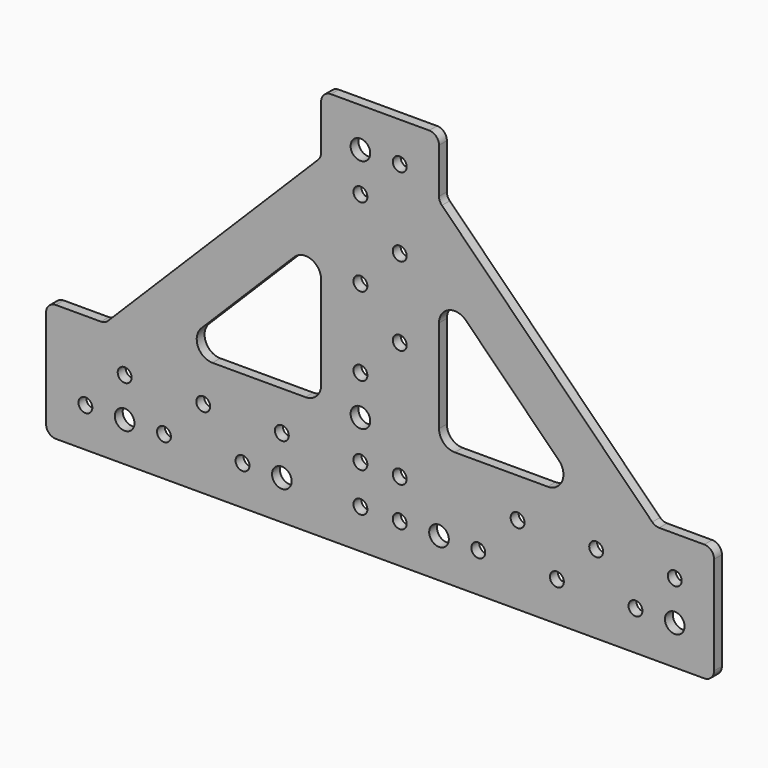
from build123d import *

# Parameters (mm, degrees)
F1_DEPTH = 3.175
F2_R     = 3.175
F3_R     = 5.08
F5_D     = 6.35
F6_D     = 4.4958
F7_R     = 5.08


with BuildPart() as f1:
    # F0 (on Front) → F1 (new body)
    with BuildSketch(Plane.XZ):
        Polygon((-25.4, 63.5), (-63.5, 63.5), (-63.5, 44.45), (-133.35, -25.4), (-152.4, -25.4), (-152.4, -63.5), (-63.5, -63.5), (63.5, -63.5), (63.5, -25.4), (44.45, -25.4), (-25.4, 44.45), align=None)
        Polygon((-63.5, 21.9964), (-63.5, -25.4), (-110.8964, -25.4), align=None, mode=Mode.SUBTRACT)
        Polygon((-25.4, -25.4), (-25.4, 21.9993596973), (21.9993596973, -25.4), align=None, mode=Mode.SUBTRACT)
    extrude(amount=F1_DEPTH)

    # F2
    f2_edges = [f1.edges().sort_by_distance(p)[0] for p in [
        (-25.4, -1.5875, 63.5),
        (-25.4, -1.5875, 44.45),
        (44.45, -1.5875, -25.4),
        (63.5, -1.5875, -25.4),
        (63.5, -1.5875, -63.5),
        (-63.5, -1.5875, 63.5),
        (-133.35, -1.5875, -25.4),
        (-152.4, -1.5875, -25.4),
        (-152.4, -1.5875, -63.5),
        (-63.5, -1.5875, 44.45),
    ]]
    fillet(f2_edges, radius=F2_R)

    # F3
    f3_edges = [f1.edges().sort_by_distance(p)[0] for p in [
        (21.99936, -1.5875, -25.4),
        (-25.4, -1.5875, -25.4),
        (-25.4, -1.5875, 21.99936),
    ]]
    fillet(f3_edges, radius=F3_R)

    # F5 (through all)
    with Locations(Plane.XZ.offset(3.175)):
        with Locations((-50.8, 50.8), (-50.8, -25.4), (50.8, -50.8), (-25.4, -50.8), (-76.2, -50.8), (-127, -50.8)):
            Hole(F5_D / 2)

    # F6 (through all)
    with Locations(Plane.XZ.offset(3.175)):
        with Locations((-50.8, 38.1), (-38.1, 50.8), (-38.1, 25.4), (-50.8, 12.7), (-38.1, 0), (-50.8, -12.7), (-38.1, -38.1), (-50.8, -38.1), (-50.8, -50.8), (-38.1, -50.8), (-12.7, -50.8), (0, -38.1), (12.7, -50.8), (25.4, -38.1), (38.1, -50.8), (50.8, -38.1), (-139.7, -50.8), (-127, -38.1), (-114.3, -50.8), (-101.6, -38.1), (-88.9, -50.8), (-76.2, -38.1)):
            Hole(F6_D / 2)

    # F7
    f7_edges = [f1.edges().sort_by_distance(p)[0] for p in [
        (-110.8964, -1.5875, -25.4),
        (-63.5, -1.5875, -25.4),
        (-63.5, -1.5875, 21.9964),
    ]]
    fillet(f7_edges, radius=F7_R)


solid = f1.part
